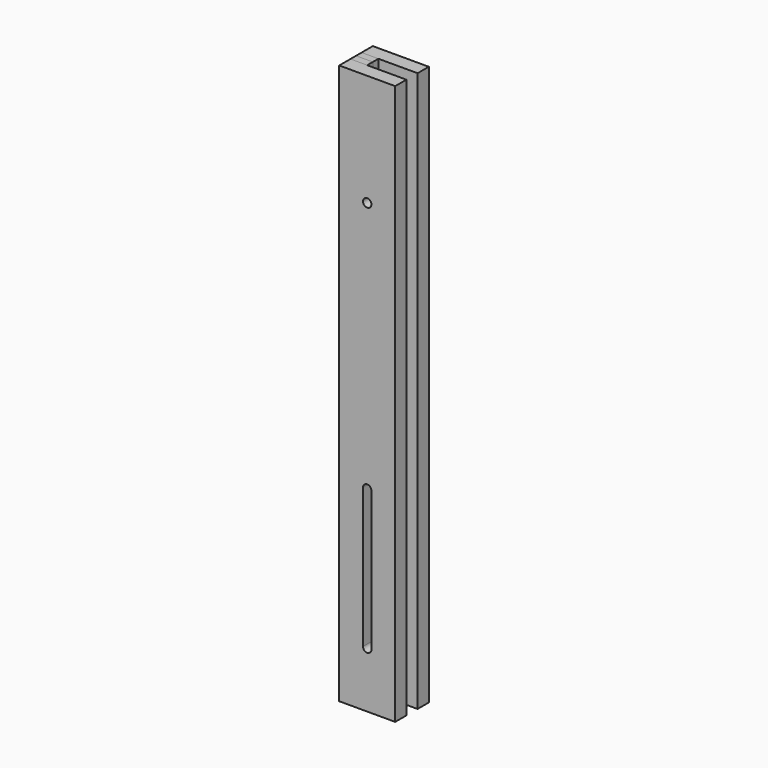
from build123d import *

# Parameters (mm, degrees)
F0_W     = 100
F0_H     = 1000
F0_R     = 7.5
F1_DEPTH = 25
F2_W     = 30
F2_H     = 12.5
F3_DEPTH = 1000


# Not quite as in the source:
# - a feature names something its author has since deleted; it is built from what else it names


with BuildPart() as f1:
    # F0 (on Front) → F1 (new body)
    with BuildSketch(Plane.XZ):
        with Locations((50, 500)):
            Rectangle(F0_W, F0_H)
        with BuildLine():
            Line((57.5, 350), (57.5, 100))
            ThreePointArc((57.5, 100), (50, 92.5), (42.5, 100))
            Line((42.5, 100), (42.5, 350))
            ThreePointArc((42.5, 350), (50, 357.5), (57.5, 350))
        make_face(mode=Mode.SUBTRACT)
        with Locations((50, 800)):
            Circle(F0_R, mode=Mode.SUBTRACT)
    extrude(amount=F1_DEPTH)


with BuildPart() as f3:
    # F2 (on face) → F3 (new body, through all)
    with BuildSketch(Plane.XY.offset(1000)):
        with Locations((15, 6.25)):
            Rectangle(F2_W, F2_H)
    extrude(amount=-F3_DEPTH)


with BuildPart() as f4_1:
    # F4: instance of F1
    add(f1.part.mirror(Plane(origin=(15, 12.5, 500), x_dir=(-1, 0, 0), z_dir=(0, 1, 0))))


with BuildPart() as f4_2:
    # F4: instance of F3
    add(f3.part.mirror(Plane(origin=(15, 12.5, 500), x_dir=(-1, 0, 0), z_dir=(0, 1, 0))))


solid = Compound([f1.part, f3.part, f4_1.part, f4_2.part])
